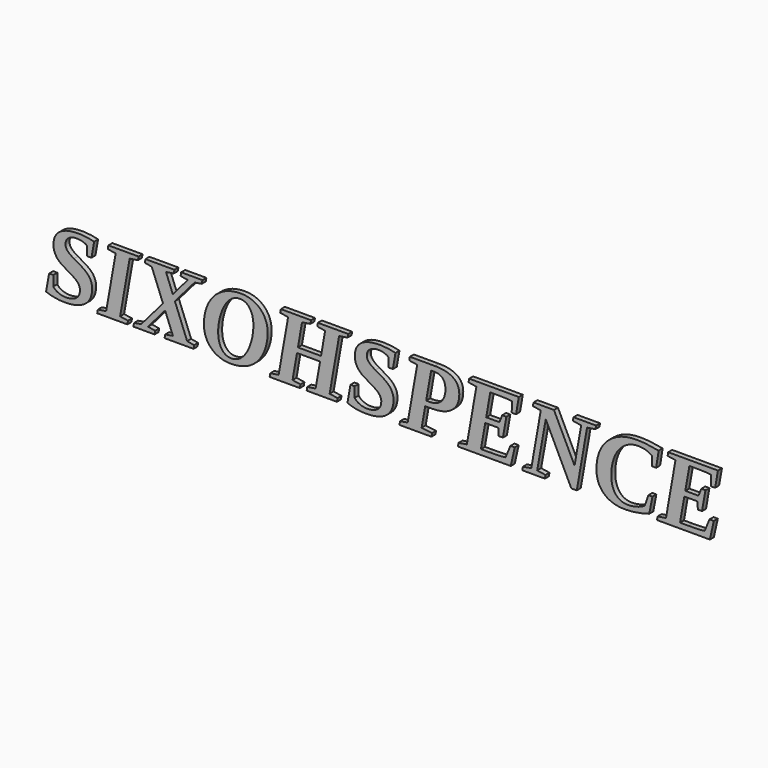
from build123d import *

# Parameters (mm, degrees)
F0_TEXT_SIZE = 49.3596618374
F1_DEPTH     = 2.54


# Not quite as in the source:
# - Text() gives the source's letters only with a copy of the font that has no kerning and outlines rounded to 1/6400 em; it was checked with that copy


with BuildPart() as f1:
    # F0 (on Front) → F1 (new body)
    with BuildSketch(Plane.XZ):
        with Locations((-64.7571980953, 0)):
            Text('SIXOHSPENCE', F0_TEXT_SIZE, font='Tinos', font_style=FontStyle.BOLDITALIC, text_align=(TextAlign.LEFT, TextAlign.BOTTOM))
    extrude(amount=F1_DEPTH)


solid = f1.part
